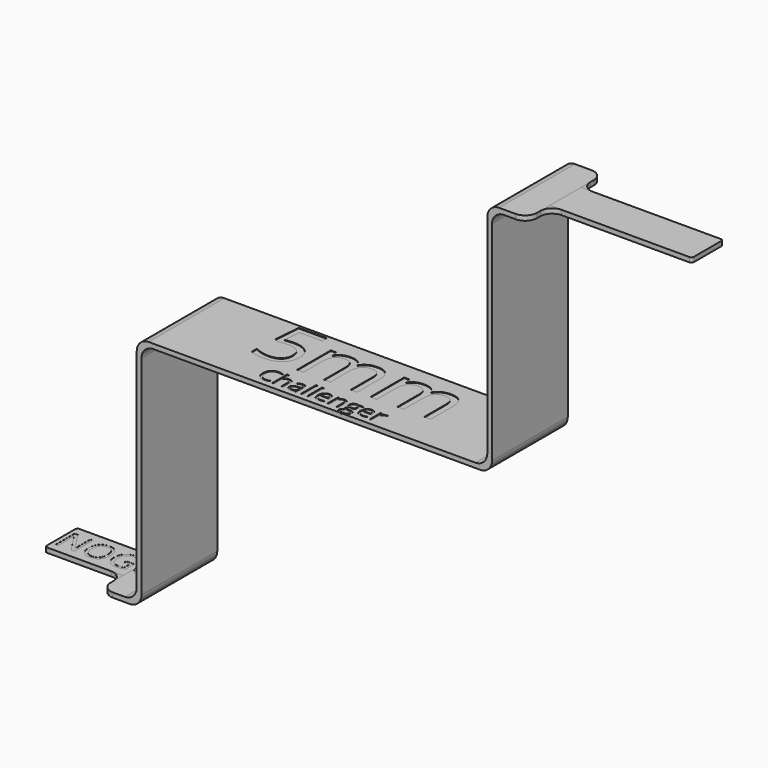
from build123d import *

# Parameters (mm, degrees)
F1_DEPTH      = 4
F0_W          = 6.6
F0_H          = 0.4
F2_DEPTH      = 1.7
F0_W_2        = 12
F3_DEPTH      = 1.65
F4_R          = 1
F5_R          = 1
F6_R          = 0.2
F6_2_R        = 0.2
F10_DEPTH     = 0.4
F12_DEPTH     = 0.4
F13_DEPTH     = 0.01
F14_TEXT_SIZE = 6.6666666667
F15_DEPTH     = 0.05
F16_TEXT_SIZE = 3.3333333333
F17_DEPTH     = 0.05
F14_W         = 0.1689453125
F14_H         = 1.5830078125
F18_DEPTH     = 0.05
F19_DEPTH     = 0.01


# Not quite as in the source:
# - Text() gives the source's letters only with a copy of the font that has no kerning and outlines rounded to 1/6400 em; it was checked with that copy


with BuildPart() as f1:
    # F0 (on Front) → F1 (new body, symmetric)
    with BuildSketch(Plane.XZ):
        Polygon((6.6, 0.4), (6.6, 0), (10, 0), (10, 19.6), (39.6, 19.6), (39.6, 39.2), (42.6, 39.2), (42.6, 39.6), (39.2, 39.6), (39.2, 20), (9.6, 20), (9.6, 0.4), align=None)
    extrude(amount=F1_DEPTH, both=True)

    # F4
    f4_edges = [f1.edges().sort_by_distance(p)[0] for p in [
        (9.6, 0, 20),
        (39.6, 0, 19.6),
        (39.2, 0, 20),
        (10, 0, 19.6),
        (39.2, 0, 39.6),
        (10, 0, 0),
        (9.6, 0, 0.4),
        (39.6, 0, 39.2),
    ]]
    fillet(f4_edges, radius=F4_R)

    # F5
    f5_edges = [f1.edges().sort_by_distance(p)[0] for p in [
        (6.6, 4, 0.2),
        (6.6, -4, 0.2),
        (42.6, -4, 39.4),
        (42.6, 4, 39.4),
    ]]
    fillet(f5_edges, radius=F5_R)


with BuildPart() as f2:
    # F0 (on Front) → F2 (new body, symmetric)
    with BuildSketch(Plane.XZ):
        with Locations((3.3, 0.2)):
            Rectangle(F0_W, F0_H)
    extrude(amount=F2_DEPTH, both=True)

    # F6
    f6_edges = [f2.edges().sort_by_distance(p)[0] for p in [
        (0, 1.7, 0.2),
        (0, -1.7, 0.2),
    ]]
    fillet(f6_edges, radius=F6_R)


with BuildPart() as f3:
    # F0 (on Front) → F3 (new body, symmetric)
    with BuildSketch(Plane.XZ):
        with Locations((48.6, 39.4)):
            Rectangle(F0_W_2, F0_H)
    extrude(amount=F3_DEPTH, both=True)

    # F6#2
    f6_2_edges = [f3.edges().sort_by_distance(p)[0] for p in [
        (54.6, 1.65, 39.4),
        (54.6, -1.65, 39.4),
    ]]
    fillet(f6_2_edges, radius=F6_2_R)

    # F16 (on face) → F17 (cut)
    with BuildSketch(Plane(origin=(0, 0, 39.2), x_dir=(1, 0, 0), z_dir=(0, 0, -1))):
        with Locations(Location((50.6, 1.2), (0, 0, -180))):
            Text('GO', F16_TEXT_SIZE, font='Open Sans', text_align=(TextAlign.LEFT, TextAlign.BOTTOM))
    extrude(amount=-F17_DEPTH, mode=Mode.SUBTRACT)


with BuildPart() as f10:
    # F9 (on face) → F10 (new body)
    with BuildSketch(Plane.XY.offset(0.4)):
        with BuildLine():
            Line((6.6, 1.7), (6.6, 2.7))
            ThreePointArc((6.6, 2.7), (6.3071067812, 1.9928932188), (5.6, 1.7))
            Line((5.6, 1.7), (6.6, 1.7))
        make_face()
    extrude(amount=-F10_DEPTH)


with BuildPart() as f10b:
    # F9 (on face) → F10, piece 2 (new body)
    with BuildSketch(Plane.XY.offset(0.4)):
        with BuildLine():
            Line((6.6, -2.7), (6.6, -1.7))
            Line((6.6, -1.7), (5.6, -1.7))
            ThreePointArc((5.6, -1.7), (6.3071067812, -1.9928932188), (6.6, -2.7))
        make_face()
    extrude(amount=-F10_DEPTH)


with BuildPart() as f12:
    # F11 (on face) → F12 (new body)
    with BuildSketch(Plane.XY.offset(39.6)):
        with BuildLine():
            Line((42.6, 1.65), (43.6, 1.65))
            ThreePointArc((43.6, 1.65), (42.8928932188, 1.9428932188), (42.6, 2.65))
            Line((42.6, 2.65), (42.6, 1.65))
        make_face()
    extrude(amount=-F12_DEPTH)


with BuildPart() as f12b:
    # F11 (on face) → F12, piece 2 (new body)
    with BuildSketch(Plane.XY.offset(39.6)):
        with BuildLine():
            Line((43.6, -1.65), (42.6, -1.65))
            Line((42.6, -1.65), (42.6, -2.65))
            ThreePointArc((42.6, -2.65), (42.8928932188, -1.9428932188), (43.6, -1.65))
        make_face()
    extrude(amount=-F12_DEPTH)


with BuildPart() as f13_tool:
    # F7 (on face) → F13 (new body)
    with BuildSketch(Plane.XY.offset(0.4)):
        with BuildLine():
            add(Edge.make_bspline(
                [(4.1881076389, -0.0056423611), (4.1881076389, -0.4817708333), (3.9472222222, -0.7545572917)],
                knots=[0, 0, 0, 1, 1, 1], degree=2))
            add(Edge.make_bspline(
                [(3.9480902778, 0.7430555556), (4.1881076389, 0.4717881944), (4.1881076389, -0.0056423611)],
                knots=[0, 0, 0, 1, 1, 1], degree=2))
            add(Edge.make_bspline(
                [(3.2805555556, 1.0143229167), (3.7080729167, 1.0143229167), (3.9480902778, 0.7430555556)],
                knots=[0, 0, 0, 1, 1, 1], degree=2))
            add(Edge.make_bspline(
                [(2.6026041667, 0.7478298611), (2.8413194444, 1.0143229167), (3.2805555556, 1.0143229167)],
                knots=[0, 0, 0, 1, 1, 1], degree=2))
            add(Edge.make_bspline(
                [(2.3638888889, -0.0030381944), (2.3638888889, 0.4813368056), (2.6026041667, 0.7478298611)],
                knots=[0, 0, 0, 1, 1, 1], degree=2))
            add(Edge.make_bspline(
                [(2.601953125, -0.7593315972), (2.3638888889, -0.4913194444), (2.3638888889, -0.0030381944)],
                knots=[0, 0, 0, 1, 1, 1], degree=2))
            add(Edge.make_bspline(
                [(3.2779513889, -1.02734375), (2.8400173611, -1.02734375), (2.601953125, -0.7593315972)],
                knots=[0, 0, 0, 1, 1, 1], degree=2))
            add(Edge.make_bspline(
                [(3.9472222222, -0.7545572917), (3.7063368056, -1.02734375), (3.2779513889, -1.02734375)],
                knots=[0, 0, 0, 1, 1, 1], degree=2))
        make_face()
        with BuildLine():
            add(Edge.make_bspline(
                [(2.6078125, -0.0056423611), (2.6078125, -0.4084201389), (2.7794704861, -0.6167534722)],
                knots=[0, 0, 0, 1, 1, 1], degree=2))
            add(Edge.make_bspline(
                [(2.7794704861, 0.5998263889), (2.6078125, 0.3914930556), (2.6078125, -0.0056423611)],
                knots=[0, 0, 0, 1, 1, 1], degree=2))
            add(Edge.make_bspline(
                [(3.2805555556, 0.8081597222), (2.9511284722, 0.8081597222), (2.7794704861, 0.5998263889)],
                knots=[0, 0, 0, 1, 1, 1], degree=2))
            add(Edge.make_bspline(
                [(3.7762152778, 0.6013454861), (3.6086805556, 0.8081597222), (3.2805555556, 0.8081597222)],
                knots=[0, 0, 0, 1, 1, 1], degree=2))
            add(Edge.make_bspline(
                [(3.94375, -0.0056423611), (3.94375, 0.39453125), (3.7762152778, 0.6013454861)],
                knots=[0, 0, 0, 1, 1, 1], degree=2))
            add(Edge.make_bspline(
                [(3.7755642361, -0.6176215278), (3.94375, -0.41015625), (3.94375, -0.0056423611)],
                knots=[0, 0, 0, 1, 1, 1], degree=2))
            add(Edge.make_bspline(
                [(3.2779513889, -0.8250868056), (3.6073784722, -0.8250868056), (3.7755642361, -0.6176215278)],
                knots=[0, 0, 0, 1, 1, 1], degree=2))
            add(Edge.make_bspline(
                [(2.7794704861, -0.6167534722), (2.9511284722, -0.8250868056), (3.2779513889, -0.8250868056)],
                knots=[0, 0, 0, 1, 1, 1], degree=2))
        make_face(mode=Mode.SUBTRACT)
        with BuildLine():
            Line((6.1763888889, 0.0390625), (5.50234375, 0.0390625))
            Line((5.50234375, 0.0390625), (5.50234375, -0.1671006944))
            Line((5.50234375, -0.1671006944), (5.9454861111, -0.1671006944))
            Line((5.9454861111, -0.1671006944), (5.9454861111, -0.77734375))
            add(Edge.make_bspline(
                [(5.5427083333, -0.8250868056), (5.7488715278, -0.8250868056), (5.9454861111, -0.77734375)],
                knots=[0, 0, 0, 1, 1, 1], degree=2))
            add(Edge.make_bspline(
                [(4.9669704861, -0.6176215278), (5.1629340278, -0.8250868056), (5.5427083333, -0.8250868056)],
                knots=[0, 0, 0, 1, 1, 1], degree=2))
            add(Edge.make_bspline(
                [(4.7710069444, -0.0086805556), (4.7710069444, -0.41015625), (4.9669704861, -0.6176215278)],
                knots=[0, 0, 0, 1, 1, 1], degree=2))
            add(Edge.make_bspline(
                [(4.9745659722, 0.5896267361), (4.7710069444, 0.3741319444), (4.7710069444, -0.0086805556)],
                knots=[0, 0, 0, 1, 1, 1], degree=2))
            add(Edge.make_bspline(
                [(5.5401041667, 0.8051215278), (5.178125, 0.8051215278), (4.9745659722, 0.5896267361)],
                knots=[0, 0, 0, 1, 1, 1], degree=2))
            add(Edge.make_bspline(
                [(6.05703125, 0.69140625), (5.7883680556, 0.8051215278), (5.5401041667, 0.8051215278)],
                knots=[0, 0, 0, 1, 1, 1], degree=2))
            Line((6.05703125, 0.69140625), (6.1464409722, 0.8949652778))
            add(Edge.make_bspline(
                [(5.5548611111, 1.0112847222), (5.8725694444, 1.0112847222), (6.1464409722, 0.8949652778)],
                knots=[0, 0, 0, 1, 1, 1], degree=2))
            add(Edge.make_bspline(
                [(5.0086371528, 0.888671875), (5.2419270833, 1.0112847222), (5.5548611111, 1.0112847222)],
                knots=[0, 0, 0, 1, 1, 1], degree=2))
            add(Edge.make_bspline(
                [(4.6512152778, 0.5334201389), (4.7753472222, 0.7660590278), (5.0086371528, 0.888671875)],
                knots=[0, 0, 0, 1, 1, 1], degree=2))
            add(Edge.make_bspline(
                [(4.5270833333, -0.0086805556), (4.5270833333, 0.30078125), (4.6512152778, 0.5334201389)],
                knots=[0, 0, 0, 1, 1, 1], degree=2))
            add(Edge.make_bspline(
                [(4.7779513889, -0.7593315972), (4.5270833333, -0.4913194444), (4.5270833333, -0.0086805556)],
                knots=[0, 0, 0, 1, 1, 1], degree=2))
            add(Edge.make_bspline(
                [(5.47890625, -1.02734375), (5.0288194444, -1.02734375), (4.7779513889, -0.7593315972)],
                knots=[0, 0, 0, 1, 1, 1], degree=2))
            add(Edge.make_bspline(
                [(5.8560763889, -1.0015190972), (5.6933159722, -1.02734375), (5.47890625, -1.02734375)],
                knots=[0, 0, 0, 1, 1, 1], degree=2))
            add(Edge.make_bspline(
                [(6.1763888889, -0.9253472222), (6.0188368056, -0.9756944444), (5.8560763889, -1.0015190972)],
                knots=[0, 0, 0, 1, 1, 1], degree=2))
            Line((6.1763888889, -0.9253472222), (6.1763888889, 0.0390625))
        make_face()
        with BuildLine():
            add(Edge.make_bspline(
                [(8.3734375, -0.0056423611), (8.3734375, -0.4817708333), (8.1325520833, -0.7545572917)],
                knots=[0, 0, 0, 1, 1, 1], degree=2))
            add(Edge.make_bspline(
                [(8.1334201389, 0.7430555556), (8.3734375, 0.4717881944), (8.3734375, -0.0056423611)],
                knots=[0, 0, 0, 1, 1, 1], degree=2))
            add(Edge.make_bspline(
                [(7.4658854167, 1.0143229167), (7.8934027778, 1.0143229167), (8.1334201389, 0.7430555556)],
                knots=[0, 0, 0, 1, 1, 1], degree=2))
            add(Edge.make_bspline(
                [(6.7879340278, 0.7478298611), (7.0266493056, 1.0143229167), (7.4658854167, 1.0143229167)],
                knots=[0, 0, 0, 1, 1, 1], degree=2))
            add(Edge.make_bspline(
                [(6.6, 0.397422803), (6.6593198862, 0.6042497104), (6.7879340278, 0.7478298611)],
                knots=[0.4612236689, 0.4612236689, 0.4612236689, 1, 1, 1], degree=2))
            Line((6.6, 0.397422803), (6.6, -0.407082007))
            add(Edge.make_bspline(
                [(6.7872829861, -0.7593315972), (6.6591696458, -0.6151019024), (6.6, -0.407082007)],
                knots=[0, 0, 0, 0.5381461004, 0.5381461004, 0.5381461004], degree=2))
            add(Edge.make_bspline(
                [(7.46328125, -1.02734375), (7.0253472222, -1.02734375), (6.7872829861, -0.7593315972)],
                knots=[0, 0, 0, 1, 1, 1], degree=2))
            add(Edge.make_bspline(
                [(8.1325520833, -0.7545572917), (7.8916666667, -1.02734375), (7.46328125, -1.02734375)],
                knots=[0, 0, 0, 1, 1, 1], degree=2))
        make_face()
        with BuildLine():
            add(Edge.make_bspline(
                [(6.7931423611, -0.0056423611), (6.7931423611, -0.4084201389), (6.9648003472, -0.6167534722)],
                knots=[0, 0, 0, 1, 1, 1], degree=2))
            add(Edge.make_bspline(
                [(6.9648003472, 0.5998263889), (6.7931423611, 0.3914930556), (6.7931423611, -0.0056423611)],
                knots=[0, 0, 0, 1, 1, 1], degree=2))
            add(Edge.make_bspline(
                [(7.4658854167, 0.8081597222), (7.1364583333, 0.8081597222), (6.9648003472, 0.5998263889)],
                knots=[0, 0, 0, 1, 1, 1], degree=2))
            add(Edge.make_bspline(
                [(7.9615451389, 0.6013454861), (7.7940104167, 0.8081597222), (7.4658854167, 0.8081597222)],
                knots=[0, 0, 0, 1, 1, 1], degree=2))
            add(Edge.make_bspline(
                [(8.1290798611, -0.0056423611), (8.1290798611, 0.39453125), (7.9615451389, 0.6013454861)],
                knots=[0, 0, 0, 1, 1, 1], degree=2))
            add(Edge.make_bspline(
                [(7.9608940972, -0.6176215278), (8.1290798611, -0.41015625), (8.1290798611, -0.0056423611)],
                knots=[0, 0, 0, 1, 1, 1], degree=2))
            add(Edge.make_bspline(
                [(7.46328125, -0.8250868056), (7.7927083333, -0.8250868056), (7.9608940972, -0.6176215278)],
                knots=[0, 0, 0, 1, 1, 1], degree=2))
            add(Edge.make_bspline(
                [(6.9648003472, -0.6167534722), (7.1364583333, -0.8250868056), (7.46328125, -0.8250868056)],
                knots=[0, 0, 0, 1, 1, 1], degree=2))
        make_face(mode=Mode.SUBTRACT)
        with BuildLine():
            Line((1.65859375, -1), (1.9216145833, -1))
            Line((1.9216145833, -1), (1.9216145833, 0.9830729167))
            Line((1.9216145833, 0.9830729167), (1.7059027778, 0.9830729167))
            Line((1.7059027778, 0.9830729167), (1.7059027778, -0.1549479167))
            add(Edge.make_bspline(
                [(1.7128472222, -0.4392361111), (1.7032986111, -0.2404513889), (1.7059027778, -0.1549479167)],
                knots=[0, 0, 0, 1, 1, 1], degree=2))
            add(Edge.make_bspline(
                [(1.725, -0.6744791667), (1.7223958333, -0.6380208333), (1.7128472222, -0.4392361111)],
                knots=[0, 0, 0, 1, 1, 1], degree=2))
            Line((1.725, -0.6744791667), (1.7141493056, -0.6744791667))
            Line((1.7141493056, -0.6744791667), (0.6329861111, 0.9830729167))
            Line((0.6329861111, 0.9830729167), (0.3725694444, 0.9830729167))
            Line((0.3725694444, 0.9830729167), (0.3725694444, -1))
            Line((0.3725694444, -1), (0.5856770833, -1))
            Line((0.5856770833, -1), (0.5856770833, 0.1271701389))
            add(Edge.make_bspline(
                [(0.5639756944, 0.6640625), (0.5856770833, 0.37109375), (0.5856770833, 0.1271701389)],
                knots=[0, 0, 0, 1, 1, 1], degree=2))
            Line((0.5639756944, 0.6640625), (0.5748263889, 0.6640625))
            Line((0.5748263889, 0.6640625), (1.65859375, -1))
        make_face()
    extrude(amount=-F13_DEPTH)


with BuildPart() as f1_1:
    add(f1.part)

    # F13: cut by f13_tool
    add(f13_tool.part, mode=Mode.SUBTRACT)

    # F14 (on face) → F15 (cut)
    with BuildSketch(Plane.XY.offset(20)):
        with Locations((16.3473958333, -1)):
            Text('5mm', F14_TEXT_SIZE, font='Open Sans', text_align=(TextAlign.LEFT, TextAlign.BOTTOM))
    extrude(amount=-F15_DEPTH, mode=Mode.SUBTRACT)

    # F14 (on face) → F18 (cut)
    with BuildSketch(Plane.XY.offset(20)):
        with BuildLine():
            add(Edge.make_bspline(
                [(19.9813802083, -2.1461588542), (19.7362630208, -2.1461588542), (19.5943359375, -2.3094075521)],
                knots=[0, 0, 0, 1, 1, 1], degree=2))
            add(Edge.make_bspline(
                [(20.3192708333, -2.2252604167), (20.1503255208, -2.1461588542), (19.9813802083, -2.1461588542)],
                knots=[0, 0, 0, 1, 1, 1], degree=2))
            Line((20.3192708333, -2.2252604167), (20.3925130208, -2.0768229167))
            add(Edge.make_bspline(
                [(19.9836588542, -1.9915364583), (20.2173828125, -1.9915364583), (20.3925130208, -2.0768229167)],
                knots=[0, 0, 0, 1, 1, 1], degree=2))
            add(Edge.make_bspline(
                [(19.6016601563, -2.0851236979), (19.7639322917, -1.9915364583), (19.9836588542, -1.9915364583)],
                knots=[0, 0, 0, 1, 1, 1], degree=2))
            add(Edge.make_bspline(
                [(19.3534505208, -2.3515625), (19.4393880208, -2.1787109375), (19.6016601563, -2.0851236979)],
                knots=[0, 0, 0, 1, 1, 1], degree=2))
            add(Edge.make_bspline(
                [(19.2675130208, -2.7542317708), (19.2675130208, -2.5244140625), (19.3534505208, -2.3515625)],
                knots=[0, 0, 0, 1, 1, 1], degree=2))
            add(Edge.make_bspline(
                [(19.4460611979, -3.3209635417), (19.2675130208, -3.1214192708), (19.2675130208, -2.7542317708)],
                knots=[0, 0, 0, 1, 1, 1], degree=2))
            add(Edge.make_bspline(
                [(19.9530598958, -3.5205078125), (19.624609375, -3.5205078125), (19.4460611979, -3.3209635417)],
                knots=[0, 0, 0, 1, 1, 1], degree=2))
            add(Edge.make_bspline(
                [(20.3345703125, -3.4622395833), (20.1799479167, -3.5205078125), (19.9530598958, -3.5205078125)],
                knots=[0, 0, 0, 1, 1, 1], degree=2))
            Line((20.3345703125, -3.4622395833), (20.3345703125, -3.3108723958))
            add(Edge.make_bspline(
                [(19.9794270833, -3.3668619792), (20.1350260417, -3.3668619792), (20.3345703125, -3.3108723958)],
                knots=[0, 0, 0, 1, 1, 1], degree=2))
            add(Edge.make_bspline(
                [(19.5892903646, -3.2075195313), (19.726171875, -3.3668619792), (19.9794270833, -3.3668619792)],
                knots=[0, 0, 0, 1, 1, 1], degree=2))
            add(Edge.make_bspline(
                [(19.4524088542, -2.7565104167), (19.4524088542, -3.0481770833), (19.5892903646, -3.2075195313)],
                knots=[0, 0, 0, 1, 1, 1], degree=2))
            add(Edge.make_bspline(
                [(19.5943359375, -2.3094075521), (19.4524088542, -2.47265625), (19.4524088542, -2.7565104167)],
                knots=[0, 0, 0, 1, 1, 1], degree=2))
        make_face()
        with BuildLine():
            Line((21.3967447917, -2.7786458333), (21.3967447917, -3.5))
            Line((21.3967447917, -3.5), (21.5656901042, -3.5))
            Line((21.5656901042, -3.5), (21.5656901042, -2.7727864583))
            add(Edge.make_bspline(
                [(21.4633138021, -2.4640299479), (21.5656901042, -2.5611979167), (21.5656901042, -2.7727864583)],
                knots=[0, 0, 0, 1, 1, 1], degree=2))
            add(Edge.make_bspline(
                [(21.1565104167, -2.3668619792), (21.3609375, -2.3668619792), (21.4633138021, -2.4640299479)],
                knots=[0, 0, 0, 1, 1, 1], degree=2))
            add(Edge.make_bspline(
                [(20.9465494792, -2.4130859375), (21.038671875, -2.3668619792), (21.1565104167, -2.3668619792)],
                knots=[0, 0, 0, 1, 1, 1], degree=2))
            add(Edge.make_bspline(
                [(20.8046223958, -2.5397135417), (20.8544270833, -2.4593098958), (20.9465494792, -2.4130859375)],
                knots=[0, 0, 0, 1, 1, 1], degree=2))
            Line((20.8046223958, -2.5397135417), (20.79453125, -2.5397135417))
            add(Edge.make_bspline(
                [(20.8026692708, -2.3961588542), (20.8026692708, -2.4827473958), (20.79453125, -2.5397135417)],
                knots=[0, 0, 0, 1, 1, 1], degree=2))
            Line((20.8026692708, -2.3961588542), (20.8026692708, -1.9169921875))
            Line((20.8026692708, -1.9169921875), (20.6337239583, -1.9169921875))
            Line((20.6337239583, -1.9169921875), (20.6337239583, -3.5))
            Line((20.6337239583, -3.5), (20.8026692708, -3.5))
            Line((20.8026692708, -3.5), (20.8026692708, -2.9169921875))
            add(Edge.make_bspline(
                [(20.8835611979, -2.6038411458), (20.8026692708, -2.6995442708), (20.8026692708, -2.9169921875)],
                knots=[0, 0, 0, 1, 1, 1], degree=2))
            add(Edge.make_bspline(
                [(21.140234375, -2.5081380208), (20.964453125, -2.5081380208), (20.8835611979, -2.6038411458)],
                knots=[0, 0, 0, 1, 1, 1], degree=2))
            add(Edge.make_bspline(
                [(21.3347330729, -2.5753580729), (21.2727213542, -2.5081380208), (21.140234375, -2.5081380208)],
                knots=[0, 0, 0, 1, 1, 1], degree=2))
            add(Edge.make_bspline(
                [(21.3967447917, -2.7786458333), (21.3967447917, -2.642578125), (21.3347330729, -2.5753580729)],
                knots=[0, 0, 0, 1, 1, 1], degree=2))
        make_face()
        with BuildLine():
            Line((22.5643880208, -3.3411458333), (22.5979166667, -3.5))
            Line((22.5979166667, -3.5), (22.7232421875, -3.5))
            Line((22.7232421875, -3.5), (22.7232421875, -2.7389322917))
            add(Edge.make_bspline(
                [(22.6270507813, -2.4552408854), (22.7232421875, -2.5436197917), (22.7232421875, -2.7389322917)],
                knots=[0, 0, 0, 1, 1, 1], degree=2))
            add(Edge.make_bspline(
                [(22.331640625, -2.3668619792), (22.530859375, -2.3668619792), (22.6270507813, -2.4552408854)],
                knots=[0, 0, 0, 1, 1, 1], degree=2))
            add(Edge.make_bspline(
                [(22.1345377604, -2.3922526042), (22.2326822917, -2.3668619792), (22.331640625, -2.3668619792)],
                knots=[0, 0, 0, 1, 1, 1], degree=2))
            add(Edge.make_bspline(
                [(21.9540364583, -2.4622395833), (22.0363932292, -2.4176432292), (22.1345377604, -2.3922526042)],
                knots=[0, 0, 0, 1, 1, 1], degree=2))
            Line((21.9540364583, -2.4622395833), (22.0061197917, -2.5914713542))
            add(Edge.make_bspline(
                [(22.3212239583, -2.5061848958), (22.1819010417, -2.5061848958), (22.0061197917, -2.5914713542)],
                knots=[0, 0, 0, 1, 1, 1], degree=2))
            add(Edge.make_bspline(
                [(22.5018880208, -2.5686848958), (22.4455729167, -2.5061848958), (22.3212239583, -2.5061848958)],
                knots=[0, 0, 0, 1, 1, 1], degree=2))
            add(Edge.make_bspline(
                [(22.558203125, -2.7623697917), (22.558203125, -2.6311848958), (22.5018880208, -2.5686848958)],
                knots=[0, 0, 0, 1, 1, 1], degree=2))
            Line((22.558203125, -2.7623697917), (22.558203125, -2.8317057292))
            Line((22.558203125, -2.8317057292), (22.3690755208, -2.837890625))
            add(Edge.make_bspline(
                [(21.8290364583, -3.1917317708), (21.8290364583, -2.8541666667), (22.3690755208, -2.837890625)],
                knots=[0, 0, 0, 1, 1, 1], degree=2))
            add(Edge.make_bspline(
                [(21.9231119792, -3.4348958333), (21.8290364583, -3.3492838542), (21.8290364583, -3.1917317708)],
                knots=[0, 0, 0, 1, 1, 1], degree=2))
            add(Edge.make_bspline(
                [(22.1828776042, -3.5205078125), (22.0171875, -3.5205078125), (21.9231119792, -3.4348958333)],
                knots=[0, 0, 0, 1, 1, 1], degree=2))
            add(Edge.make_bspline(
                [(22.3900716146, -3.4832356771), (22.3072265625, -3.5205078125), (22.1828776042, -3.5205078125)],
                knots=[0, 0, 0, 1, 1, 1], degree=2))
            add(Edge.make_bspline(
                [(22.55625, -3.3411458333), (22.4729166667, -3.4459635417), (22.3900716146, -3.4832356771)],
                knots=[0, 0, 0, 1, 1, 1], degree=2))
            Line((22.55625, -3.3411458333), (22.5643880208, -3.3411458333))
        make_face()
        with BuildLine():
            add(Edge.make_bspline(
                [(22.21640625, -3.380859375), (22.3742838542, -3.380859375), (22.4642903646, -3.2944335938)],
                knots=[0, 0, 0, 1, 1, 1], degree=2))
            add(Edge.make_bspline(
                [(22.0614583333, -3.3331705729), (22.116796875, -3.380859375), (22.21640625, -3.380859375)],
                knots=[0, 0, 0, 1, 1, 1], degree=2))
            add(Edge.make_bspline(
                [(22.0061197917, -3.1936848958), (22.0061197917, -3.2854817708), (22.0614583333, -3.3331705729)],
                knots=[0, 0, 0, 1, 1, 1], degree=2))
            add(Edge.make_bspline(
                [(22.0949869792, -3.0213216146), (22.0061197917, -3.0768229167), (22.0061197917, -3.1936848958)],
                knots=[0, 0, 0, 1, 1, 1], degree=2))
            add(Edge.make_bspline(
                [(22.3853515625, -2.9586588542), (22.1838541667, -2.9658203125), (22.0949869792, -3.0213216146)],
                knots=[0, 0, 0, 1, 1, 1], degree=2))
            Line((22.3853515625, -2.9586588542), (22.554296875, -2.9518229167))
            Line((22.554296875, -2.9518229167), (22.554296875, -3.0524088542))
            add(Edge.make_bspline(
                [(22.4642903646, -3.2944335938), (22.554296875, -3.2080078125), (22.554296875, -3.0524088542)],
                knots=[0, 0, 0, 1, 1, 1], degree=2))
        make_face(mode=Mode.SUBTRACT)
        with Locations((23.1553710938, -2.7084960938)):
            Rectangle(F14_W, F14_H)
        with Locations((23.6823893229, -2.7084960938)):
            Rectangle(F14_W, F14_H)
        with BuildLine():
            add(Edge.make_bspline(
                [(24.5959635417, -3.5205078125), (24.3488932292, -3.5205078125), (24.2058268229, -3.3697916667)],
                knots=[0, 0, 0, 1, 1, 1], degree=2))
            add(Edge.make_bspline(
                [(24.788671875, -3.5035807292), (24.7089192708, -3.5205078125), (24.5959635417, -3.5205078125)],
                knots=[0, 0, 0, 1, 1, 1], degree=2))
            add(Edge.make_bspline(
                [(24.9579427083, -3.4482421875), (24.8684244792, -3.4866536458), (24.788671875, -3.5035807292)],
                knots=[0, 0, 0, 1, 1, 1], degree=2))
            Line((24.9579427083, -3.4482421875), (24.9579427083, -3.2975260417))
            add(Edge.make_bspline(
                [(24.6021484375, -3.3727213542), (24.7821614583, -3.3727213542), (24.9579427083, -3.2975260417)],
                knots=[0, 0, 0, 1, 1, 1], degree=2))
            add(Edge.make_bspline(
                [(24.3371744792, -3.2709960938), (24.43125, -3.3727213542), (24.6021484375, -3.3727213542)],
                knots=[0, 0, 0, 1, 1, 1], degree=2))
            add(Edge.make_bspline(
                [(24.237890625, -2.9729817708), (24.2430989583, -3.1692708333), (24.3371744792, -3.2709960938)],
                knots=[0, 0, 0, 1, 1, 1], degree=2))
            Line((24.237890625, -2.9729817708), (25.0057942708, -2.9729817708))
            Line((25.0057942708, -2.9729817708), (25.0057942708, -2.8662109375))
            add(Edge.make_bspline(
                [(24.8837239583, -2.5024414063), (25.0057942708, -2.6402994792), (25.0057942708, -2.8662109375)],
                knots=[0, 0, 0, 1, 1, 1], degree=2))
            add(Edge.make_bspline(
                [(24.55234375, -2.3645833333), (24.7616536458, -2.3645833333), (24.8837239583, -2.5024414063)],
                knots=[0, 0, 0, 1, 1, 1], degree=2))
            add(Edge.make_bspline(
                [(24.1955729167, -2.5232747396), (24.3283854167, -2.3645833333), (24.55234375, -2.3645833333)],
                knots=[0, 0, 0, 1, 1, 1], degree=2))
            add(Edge.make_bspline(
                [(24.0627604167, -2.9518229167), (24.0627604167, -2.6819661458), (24.1955729167, -2.5232747396)],
                knots=[0, 0, 0, 1, 1, 1], degree=2))
            add(Edge.make_bspline(
                [(24.2058268229, -3.3697916667), (24.0627604167, -3.2190755208), (24.0627604167, -2.9518229167)],
                knots=[0, 0, 0, 1, 1, 1], degree=2))
        make_face()
        with BuildLine():
            add(Edge.make_bspline(
                [(24.5500651042, -2.5061848958), (24.4159505208, -2.5061848958), (24.3360351563, -2.5935872396)],
                knots=[0, 0, 0, 1, 1, 1], degree=2))
            add(Edge.make_bspline(
                [(24.7536783854, -2.5911458333), (24.6825520833, -2.5061848958), (24.5500651042, -2.5061848958)],
                knots=[0, 0, 0, 1, 1, 1], degree=2))
            add(Edge.make_bspline(
                [(24.8248046875, -2.8356119792), (24.8248046875, -2.6761067708), (24.7536783854, -2.5911458333)],
                knots=[0, 0, 0, 1, 1, 1], degree=2))
            Line((24.8248046875, -2.8356119792), (24.241796875, -2.8356119792))
            add(Edge.make_bspline(
                [(24.3360351563, -2.5935872396), (24.2561197917, -2.6809895833), (24.241796875, -2.8356119792)],
                knots=[0, 0, 0, 1, 1, 1], degree=2))
        make_face(mode=Mode.SUBTRACT)
        with BuildLine():
            Line((26.0569010417, -2.7786458333), (26.0569010417, -3.5))
            Line((26.0569010417, -3.5), (26.2258463542, -3.5))
            Line((26.2258463542, -3.5), (26.2258463542, -2.7727864583))
            add(Edge.make_bspline(
                [(26.1241210938, -2.4617513021), (26.2258463542, -2.5589192708), (26.2258463542, -2.7727864583)],
                knots=[0, 0, 0, 1, 1, 1], degree=2))
            add(Edge.make_bspline(
                [(25.8208984375, -2.3645833333), (26.0223958333, -2.3645833333), (26.1241210938, -2.4617513021)],
                knots=[0, 0, 0, 1, 1, 1], degree=2))
            add(Edge.make_bspline(
                [(25.6124023438, -2.4099934896), (25.7059895833, -2.3645833333), (25.8208984375, -2.3645833333)],
                knots=[0, 0, 0, 1, 1, 1], degree=2))
            add(Edge.make_bspline(
                [(25.4667317708, -2.5377604167), (25.5188151042, -2.4554036458), (25.6124023438, -2.4099934896)],
                knots=[0, 0, 0, 1, 1, 1], degree=2))
            Line((25.4667317708, -2.5377604167), (25.45859375, -2.5377604167))
            Line((25.45859375, -2.5377604167), (25.43125, -2.3850911458))
            Line((25.43125, -2.3850911458), (25.2938802083, -2.3850911458))
            Line((25.2938802083, -2.3850911458), (25.2938802083, -3.5))
            Line((25.2938802083, -3.5), (25.4628255208, -3.5))
            Line((25.4628255208, -3.5), (25.4628255208, -2.9150390625))
            add(Edge.make_bspline(
                [(25.5442057292, -2.6027018229), (25.4628255208, -2.697265625), (25.4628255208, -2.9150390625)],
                knots=[0, 0, 0, 1, 1, 1], degree=2))
            add(Edge.make_bspline(
                [(25.800390625, -2.5081380208), (25.6255859375, -2.5081380208), (25.5442057292, -2.6027018229)],
                knots=[0, 0, 0, 1, 1, 1], degree=2))
            add(Edge.make_bspline(
                [(25.9948893229, -2.5753580729), (25.9328776042, -2.5081380208), (25.800390625, -2.5081380208)],
                knots=[0, 0, 0, 1, 1, 1], degree=2))
            add(Edge.make_bspline(
                [(26.0569010417, -2.7786458333), (26.0569010417, -2.642578125), (25.9948893229, -2.5753580729)],
                knots=[0, 0, 0, 1, 1, 1], degree=2))
        make_face()
        with BuildLine():
            add(Edge.make_bspline(
                [(26.8506031854, -4), (26.6595842611, -3.9933721746), (26.5516927083, -3.9192708333)],
                knots=[0.0894427191, 0.0894427191, 0.0894427191, 1, 1, 1], degree=2))
            Line((26.8506031854, -4), (26.934647817, -4))
            add(Edge.make_bspline(
                [(27.3222005208, -3.9034830729), (27.1859133057, -3.9926974012), (26.934647817, -4)],
                knots=[0, 0, 0, 0.9181454491, 0.9181454491, 0.9181454491], degree=2))
            add(Edge.make_bspline(
                [(27.4706380208, -3.62109375), (27.4706380208, -3.8063151042), (27.3222005208, -3.9034830729)],
                knots=[0, 0, 0, 1, 1, 1], degree=2))
            add(Edge.make_bspline(
                [(27.3736328125, -3.3992513021), (27.4706380208, -3.4755859375), (27.4706380208, -3.62109375)],
                knots=[0, 0, 0, 1, 1, 1], degree=2))
            add(Edge.make_bspline(
                [(27.0953125, -3.3229166667), (27.2766276042, -3.3229166667), (27.3736328125, -3.3992513021)],
                knots=[0, 0, 0, 1, 1, 1], degree=2))
            Line((27.0953125, -3.3229166667), (26.898046875, -3.3229166667))
            add(Edge.make_bspline(
                [(26.7689778646, -3.3011067708), (26.8065755208, -3.3229166667), (26.898046875, -3.3229166667)],
                knots=[0, 0, 0, 1, 1, 1], degree=2))
            add(Edge.make_bspline(
                [(26.7313802083, -3.2333984375), (26.7313802083, -3.279296875), (26.7689778646, -3.3011067708)],
                knots=[0, 0, 0, 1, 1, 1], degree=2))
            add(Edge.make_bspline(
                [(26.8391276042, -3.0901692708), (26.7313802083, -3.1471354167), (26.7313802083, -3.2333984375)],
                knots=[0, 0, 0, 1, 1, 1], degree=2))
            add(Edge.make_bspline(
                [(26.9325520833, -3.0983072917), (26.8827473958, -3.0983072917), (26.8391276042, -3.0901692708)],
                knots=[0, 0, 0, 1, 1, 1], degree=2))
            add(Edge.make_bspline(
                [(27.23984375, -3.0006510417), (27.1278645833, -3.0983072917), (26.9325520833, -3.0983072917)],
                knots=[0, 0, 0, 1, 1, 1], degree=2))
            add(Edge.make_bspline(
                [(27.3518229167, -2.7389322917), (27.3518229167, -2.9029947917), (27.23984375, -3.0006510417)],
                knots=[0, 0, 0, 1, 1, 1], degree=2))
            add(Edge.make_bspline(
                [(27.3293619792, -2.609375), (27.3518229167, -2.6669921875), (27.3518229167, -2.7389322917)],
                knots=[0, 0, 0, 1, 1, 1], degree=2))
            add(Edge.make_bspline(
                [(27.2785807292, -2.5162760417), (27.3069010417, -2.5517578125), (27.3293619792, -2.609375)],
                knots=[0, 0, 0, 1, 1, 1], degree=2))
            Line((27.2785807292, -2.5162760417), (27.4849609375, -2.4918619792))
            Line((27.4849609375, -2.4918619792), (27.4849609375, -2.3850911458))
            Line((27.4849609375, -2.3850911458), (27.0995442708, -2.3850911458))
            add(Edge.make_bspline(
                [(26.9416666667, -2.3645833333), (27.0292317708, -2.3645833333), (27.0995442708, -2.3850911458)],
                knots=[0, 0, 0, 1, 1, 1], degree=2))
            add(Edge.make_bspline(
                [(26.6306315104, -2.4638671875), (26.7404947917, -2.3645833333), (26.9416666667, -2.3645833333)],
                knots=[0, 0, 0, 1, 1, 1], degree=2))
            add(Edge.make_bspline(
                [(26.5207682292, -2.74609375), (26.5207682292, -2.5631510417), (26.6306315104, -2.4638671875)],
                knots=[0, 0, 0, 1, 1, 1], degree=2))
            add(Edge.make_bspline(
                [(26.5751302083, -2.9415690104), (26.5207682292, -2.8561197917), (26.5207682292, -2.74609375)],
                knots=[0, 0, 0, 1, 1, 1], degree=2))
            add(Edge.make_bspline(
                [(26.7160807292, -3.0625), (26.6294921875, -3.0270182292), (26.5751302083, -2.9415690104)],
                knots=[0, 0, 0, 1, 1, 1], degree=2))
            add(Edge.make_bspline(
                [(26.6132161458, -3.1510416667), (26.6457682292, -3.1051432292), (26.7160807292, -3.0625)],
                knots=[0, 0, 0, 1, 1, 1], degree=2))
            add(Edge.make_bspline(
                [(26.5806640625, -3.2578125), (26.5806640625, -3.1969401042), (26.6132161458, -3.1510416667)],
                knots=[0, 0, 0, 1, 1, 1], degree=2))
            add(Edge.make_bspline(
                [(26.6096354167, -3.3525390625), (26.5806640625, -3.3118489583), (26.5806640625, -3.2578125)],
                knots=[0, 0, 0, 1, 1, 1], degree=2))
            add(Edge.make_bspline(
                [(26.68125, -3.4124348958), (26.6386067708, -3.3932291667), (26.6096354167, -3.3525390625)],
                knots=[0, 0, 0, 1, 1, 1], degree=2))
            add(Edge.make_bspline(
                [(26.4983072917, -3.5131835938), (26.5634114583, -3.4388020833), (26.68125, -3.4124348958)],
                knots=[0, 0, 0, 1, 1, 1], degree=2))
            add(Edge.make_bspline(
                [(26.433203125, -3.6891276042), (26.433203125, -3.5875651042), (26.4983072917, -3.5131835938)],
                knots=[0, 0, 0, 1, 1, 1], degree=2))
            add(Edge.make_bspline(
                [(26.5516927083, -3.9192708333), (26.433203125, -3.837890625), (26.433203125, -3.6891276042)],
                knots=[0, 0, 0, 1, 1, 1], degree=2))
        make_face()
        with BuildLine():
            add(Edge.make_bspline(
                [(26.5959635417, -3.6871744792), (26.5959635417, -3.7776692708), (26.6722981771, -3.8245442708)],
                knots=[0, 0, 0, 1, 1, 1], degree=2))
            add(Edge.make_bspline(
                [(26.6600911458, -3.5294596354), (26.5959635417, -3.5843098958), (26.5959635417, -3.6871744792)],
                knots=[0, 0, 0, 1, 1, 1], degree=2))
            add(Edge.make_bspline(
                [(26.8391276042, -3.474609375), (26.72421875, -3.474609375), (26.6600911458, -3.5294596354)],
                knots=[0, 0, 0, 1, 1, 1], degree=2))
            Line((26.8391276042, -3.474609375), (27.0416015625, -3.474609375))
            add(Edge.make_bspline(
                [(27.2520507813, -3.509765625), (27.1962239583, -3.474609375), (27.0416015625, -3.474609375)],
                knots=[0, 0, 0, 1, 1, 1], degree=2))
            add(Edge.make_bspline(
                [(27.3078776042, -3.6354166667), (27.3078776042, -3.544921875), (27.2520507813, -3.509765625)],
                knots=[0, 0, 0, 1, 1, 1], degree=2))
            add(Edge.make_bspline(
                [(27.2056640625, -3.8077799479), (27.3078776042, -3.744140625), (27.3078776042, -3.6354166667)],
                knots=[0, 0, 0, 1, 1, 1], degree=2))
            add(Edge.make_bspline(
                [(26.8908854167, -3.8714192708), (27.1034505208, -3.8714192708), (27.2056640625, -3.8077799479)],
                knots=[0, 0, 0, 1, 1, 1], degree=2))
            add(Edge.make_bspline(
                [(26.6722981771, -3.8245442708), (26.7486328125, -3.8714192708), (26.8908854167, -3.8714192708)],
                knots=[0, 0, 0, 1, 1, 1], degree=2))
        make_face(mode=Mode.SUBTRACT)
        with BuildLine():
            add(Edge.make_bspline(
                [(26.6874348958, -2.7421875), (26.6874348958, -2.8590494792), (26.753515625, -2.9191080729)],
                knots=[0, 0, 0, 1, 1, 1], degree=2))
            add(Edge.make_bspline(
                [(26.7515625, -2.5519205729), (26.6874348958, -2.6158854167), (26.6874348958, -2.7421875)],
                knots=[0, 0, 0, 1, 1, 1], degree=2))
            add(Edge.make_bspline(
                [(26.9348307292, -2.4879557292), (26.8156901042, -2.4879557292), (26.7515625, -2.5519205729)],
                knots=[0, 0, 0, 1, 1, 1], degree=2))
            add(Edge.make_bspline(
                [(27.1848307292, -2.7389322917), (27.1848307292, -2.4879557292), (26.9348307292, -2.4879557292)],
                knots=[0, 0, 0, 1, 1, 1], degree=2))
            add(Edge.make_bspline(
                [(26.9377604167, -2.9791666667), (27.1848307292, -2.9791666667), (27.1848307292, -2.7389322917)],
                knots=[0, 0, 0, 1, 1, 1], degree=2))
            add(Edge.make_bspline(
                [(26.753515625, -2.9191080729), (26.8195963542, -2.9791666667), (26.9377604167, -2.9791666667)],
                knots=[0, 0, 0, 1, 1, 1], degree=2))
        make_face(mode=Mode.SUBTRACT)
        with BuildLine():
            add(Edge.make_bspline(
                [(28.1848307292, -3.5205078125), (27.9377604167, -3.5205078125), (27.7946940104, -3.3697916667)],
                knots=[0, 0, 0, 1, 1, 1], degree=2))
            add(Edge.make_bspline(
                [(28.3775390625, -3.5035807292), (28.2977864583, -3.5205078125), (28.1848307292, -3.5205078125)],
                knots=[0, 0, 0, 1, 1, 1], degree=2))
            add(Edge.make_bspline(
                [(28.5468098958, -3.4482421875), (28.4572916667, -3.4866536458), (28.3775390625, -3.5035807292)],
                knots=[0, 0, 0, 1, 1, 1], degree=2))
            Line((28.5468098958, -3.4482421875), (28.5468098958, -3.2975260417))
            add(Edge.make_bspline(
                [(28.191015625, -3.3727213542), (28.3710286458, -3.3727213542), (28.5468098958, -3.2975260417)],
                knots=[0, 0, 0, 1, 1, 1], degree=2))
            add(Edge.make_bspline(
                [(27.9260416667, -3.2709960938), (28.0201171875, -3.3727213542), (28.191015625, -3.3727213542)],
                knots=[0, 0, 0, 1, 1, 1], degree=2))
            add(Edge.make_bspline(
                [(27.8267578125, -2.9729817708), (27.8319661458, -3.1692708333), (27.9260416667, -3.2709960938)],
                knots=[0, 0, 0, 1, 1, 1], degree=2))
            Line((27.8267578125, -2.9729817708), (28.5946614583, -2.9729817708))
            Line((28.5946614583, -2.9729817708), (28.5946614583, -2.8662109375))
            add(Edge.make_bspline(
                [(28.4725911458, -2.5024414063), (28.5946614583, -2.6402994792), (28.5946614583, -2.8662109375)],
                knots=[0, 0, 0, 1, 1, 1], degree=2))
            add(Edge.make_bspline(
                [(28.1412109375, -2.3645833333), (28.3505208333, -2.3645833333), (28.4725911458, -2.5024414063)],
                knots=[0, 0, 0, 1, 1, 1], degree=2))
            add(Edge.make_bspline(
                [(27.7844401042, -2.5232747396), (27.9172526042, -2.3645833333), (28.1412109375, -2.3645833333)],
                knots=[0, 0, 0, 1, 1, 1], degree=2))
            add(Edge.make_bspline(
                [(27.6516276042, -2.9518229167), (27.6516276042, -2.6819661458), (27.7844401042, -2.5232747396)],
                knots=[0, 0, 0, 1, 1, 1], degree=2))
            add(Edge.make_bspline(
                [(27.7946940104, -3.3697916667), (27.6516276042, -3.2190755208), (27.6516276042, -2.9518229167)],
                knots=[0, 0, 0, 1, 1, 1], degree=2))
        make_face()
        with BuildLine():
            add(Edge.make_bspline(
                [(28.1389322917, -2.5061848958), (28.0048177083, -2.5061848958), (27.9249023438, -2.5935872396)],
                knots=[0, 0, 0, 1, 1, 1], degree=2))
            add(Edge.make_bspline(
                [(28.3425455729, -2.5911458333), (28.2714192708, -2.5061848958), (28.1389322917, -2.5061848958)],
                knots=[0, 0, 0, 1, 1, 1], degree=2))
            add(Edge.make_bspline(
                [(28.413671875, -2.8356119792), (28.413671875, -2.6761067708), (28.3425455729, -2.5911458333)],
                knots=[0, 0, 0, 1, 1, 1], degree=2))
            Line((28.413671875, -2.8356119792), (27.8306640625, -2.8356119792))
            add(Edge.make_bspline(
                [(27.9249023438, -2.5935872396), (27.8449869792, -2.6809895833), (27.8306640625, -2.8356119792)],
                knots=[0, 0, 0, 1, 1, 1], degree=2))
        make_face(mode=Mode.SUBTRACT)
        with BuildLine():
            add(Edge.make_bspline(
                [(29.3915364583, -2.3645833333), (29.4657552083, -2.3645833333), (29.5246744792, -2.376953125)],
                knots=[0, 0, 0, 1, 1, 1], degree=2))
            add(Edge.make_bspline(
                [(29.1991536458, -2.4236653646), (29.28671875, -2.3645833333), (29.3915364583, -2.3645833333)],
                knots=[0, 0, 0, 1, 1, 1], degree=2))
            add(Edge.make_bspline(
                [(29.0497395833, -2.5914713542), (29.1115885417, -2.4827473958), (29.1991536458, -2.4236653646)],
                knots=[0, 0, 0, 1, 1, 1], degree=2))
            Line((29.0497395833, -2.5914713542), (29.0416015625, -2.5914713542))
            Line((29.0416015625, -2.5914713542), (29.0220703125, -2.3850911458))
            Line((29.0220703125, -2.3850911458), (28.8827473958, -2.3850911458))
            Line((28.8827473958, -2.3850911458), (28.8827473958, -3.5))
            Line((28.8827473958, -3.5), (29.0516927083, -3.5))
            Line((29.0516927083, -3.5), (29.0516927083, -2.9016927083))
            add(Edge.make_bspline(
                [(29.1477213542, -2.6280924479), (29.0516927083, -2.7379557292), (29.0516927083, -2.9016927083)],
                knots=[0, 0, 0, 1, 1, 1], degree=2))
            add(Edge.make_bspline(
                [(29.3791666667, -2.5182291667), (29.24375, -2.5182291667), (29.1477213542, -2.6280924479)],
                knots=[0, 0, 0, 1, 1, 1], degree=2))
            add(Edge.make_bspline(
                [(29.5012369792, -2.5335286458), (29.4322265625, -2.5182291667), (29.3791666667, -2.5182291667)],
                knots=[0, 0, 0, 1, 1, 1], degree=2))
            Line((29.5012369792, -2.5335286458), (29.5246744792, -2.376953125))
        make_face()
    extrude(amount=-F18_DEPTH, mode=Mode.SUBTRACT)

    # F7 (on face) → F19 (cut)
    with BuildSketch(Plane.XY.offset(0.4)):
        with BuildLine():
            add(Edge.make_bspline(
                [(8.3734375, -0.0056423611), (8.3734375, -0.4817708333), (8.1325520833, -0.7545572917)],
                knots=[0, 0, 0, 1, 1, 1], degree=2))
            add(Edge.make_bspline(
                [(8.1334201389, 0.7430555556), (8.3734375, 0.4717881944), (8.3734375, -0.0056423611)],
                knots=[0, 0, 0, 1, 1, 1], degree=2))
            add(Edge.make_bspline(
                [(7.4658854167, 1.0143229167), (7.8934027778, 1.0143229167), (8.1334201389, 0.7430555556)],
                knots=[0, 0, 0, 1, 1, 1], degree=2))
            add(Edge.make_bspline(
                [(6.7879340278, 0.7478298611), (7.0266493056, 1.0143229167), (7.4658854167, 1.0143229167)],
                knots=[0, 0, 0, 1, 1, 1], degree=2))
            add(Edge.make_bspline(
                [(6.6, 0.397422803), (6.6593198862, 0.6042497104), (6.7879340278, 0.7478298611)],
                knots=[0.4612236689, 0.4612236689, 0.4612236689, 1, 1, 1], degree=2))
            Line((6.6, 0.397422803), (6.6, -0.407082007))
            add(Edge.make_bspline(
                [(6.7872829861, -0.7593315972), (6.6591696458, -0.6151019024), (6.6, -0.407082007)],
                knots=[0, 0, 0, 0.5381461004, 0.5381461004, 0.5381461004], degree=2))
            add(Edge.make_bspline(
                [(7.46328125, -1.02734375), (7.0253472222, -1.02734375), (6.7872829861, -0.7593315972)],
                knots=[0, 0, 0, 1, 1, 1], degree=2))
            add(Edge.make_bspline(
                [(8.1325520833, -0.7545572917), (7.8916666667, -1.02734375), (7.46328125, -1.02734375)],
                knots=[0, 0, 0, 1, 1, 1], degree=2))
        make_face()
        with BuildLine():
            add(Edge.make_bspline(
                [(6.7931423611, -0.0056423611), (6.7931423611, -0.4084201389), (6.9648003472, -0.6167534722)],
                knots=[0, 0, 0, 1, 1, 1], degree=2))
            add(Edge.make_bspline(
                [(6.9648003472, 0.5998263889), (6.7931423611, 0.3914930556), (6.7931423611, -0.0056423611)],
                knots=[0, 0, 0, 1, 1, 1], degree=2))
            add(Edge.make_bspline(
                [(7.4658854167, 0.8081597222), (7.1364583333, 0.8081597222), (6.9648003472, 0.5998263889)],
                knots=[0, 0, 0, 1, 1, 1], degree=2))
            add(Edge.make_bspline(
                [(7.9615451389, 0.6013454861), (7.7940104167, 0.8081597222), (7.4658854167, 0.8081597222)],
                knots=[0, 0, 0, 1, 1, 1], degree=2))
            add(Edge.make_bspline(
                [(8.1290798611, -0.0056423611), (8.1290798611, 0.39453125), (7.9615451389, 0.6013454861)],
                knots=[0, 0, 0, 1, 1, 1], degree=2))
            add(Edge.make_bspline(
                [(7.9608940972, -0.6176215278), (8.1290798611, -0.41015625), (8.1290798611, -0.0056423611)],
                knots=[0, 0, 0, 1, 1, 1], degree=2))
            add(Edge.make_bspline(
                [(7.46328125, -0.8250868056), (7.7927083333, -0.8250868056), (7.9608940972, -0.6176215278)],
                knots=[0, 0, 0, 1, 1, 1], degree=2))
            add(Edge.make_bspline(
                [(6.9648003472, -0.6167534722), (7.1364583333, -0.8250868056), (7.46328125, -0.8250868056)],
                knots=[0, 0, 0, 1, 1, 1], degree=2))
        make_face(mode=Mode.SUBTRACT)
    extrude(amount=-F19_DEPTH, mode=Mode.SUBTRACT)


with BuildPart() as f2_1:
    add(f2.part)

    # F13: cut by f13_tool
    add(f13_tool.part, mode=Mode.SUBTRACT)


solid = Compound([f3.part, f10.part, f10b.part, f12.part, f12b.part, f1_1.part, f2_1.part])
